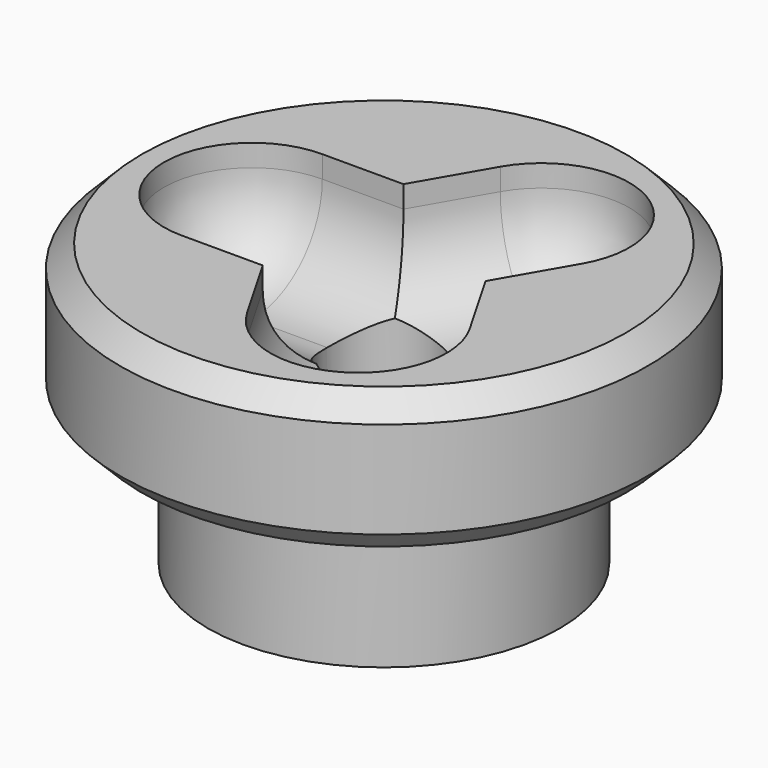
from build123d import *

# Parameters (mm, degrees)
F2_SIZE  = 0.79375
F4_DEPTH = 3.96875
F5_R     = 3.17499
F7_D     = 4.0894


# Not quite as in the source:
# - a fillet or chamfer is up to 0.001 mm smaller than in the source, because OpenCascade refuses the exact size


with BuildPart() as f1:
    # F0 (on Front) → F1 (revolve)
    with BuildSketch(Plane.XZ):
        Polygon((-6.35, -10.16), (0, -10.16), (0, 0), (-9.525, 0), (-9.525, -5.08), (-6.35, -5.08), align=None)
    revolve(axis=Axis((0, 0, -1.025330542), (0, 0, -1)))

    # F2
    f2_edges = [f1.edges().sort_by_distance(p)[0] for p in [
        (9.525, 0, 0),
        (9.525, 0, -5.08),
    ]]
    chamfer(f2_edges, length=F2_SIZE)

    # F3 (on face) → F4 (cut)
    with BuildSketch(Plane.XY):
        with BuildLine():
            Line((-4.7625, -3.175), (-1.8330871047, -3.175))
            Line((-1.8330871047, -3.175), (-0.368380657, -5.7119459855))
            ThreePointArc((-0.368380657, -5.7119459855), (3.96875, -6.8740766425), (5.130880657, -2.5369459855))
            Line((5.130880657, -2.5369459855), (3.6661742094, 0))
            Line((3.6661742094, 0), (5.130880657, 2.5369459855))
            ThreePointArc((5.130880657, 2.5369459855), (3.96875, 6.8740766425), (-0.368380657, 5.7119459855))
            Line((-0.368380657, 5.7119459855), (-1.8330871047, 3.175))
            Line((-1.8330871047, 3.175), (-4.7625, 3.175))
            ThreePointArc((-4.7625, 3.175), (-7.9375, 0), (-4.7625, -3.175))
        make_face()
    extrude(amount=-F4_DEPTH, mode=Mode.SUBTRACT)

    # F5 (radius 3.175 in the source; OpenCascade refuses exactly that, so slightly less here)
    f5_edges = [f1.edges().sort_by_distance(p)[0] for p in [
        (3.96875, 6.874077, -3.96875),
        (-1.100734, 4.443473, -3.96875),
        (-3.297794, 3.175, -3.96875),
        (-7.9375, 0, -3.96875),
        (-3.297794, -3.175, -3.96875),
        (-1.100734, -4.443473, -3.96875),
        (3.96875, -6.874077, -3.96875),
        (4.398527, -1.268473, -3.96875),
        (4.398527, 1.268473, -3.96875),
    ]]
    fillet(f5_edges, radius=F5_R)

    # F7 (through all)
    with Locations(Plane(origin=(0, 0, -10.16), x_dir=(1, 0, 0), z_dir=(0, 0, -1))):
        with Locations((0, 0)):
            Hole(F7_D / 2)


solid = f1.part
